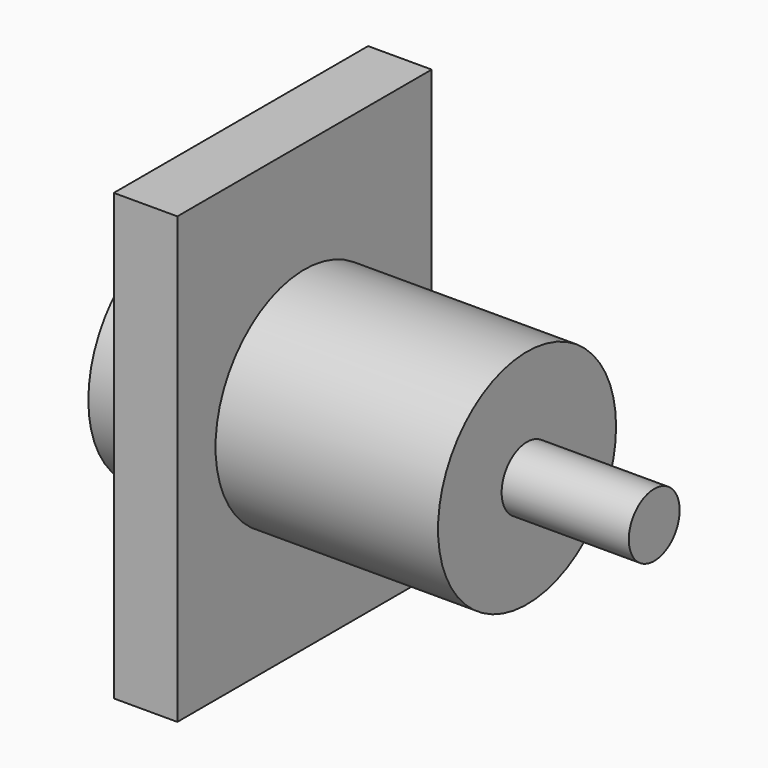
from build123d import *

# Parameters (mm, degrees)
F0_R     = 35
F1_DEPTH = 70
F2_R     = 10
F3_DEPTH = 40
F4_W     = 100
F4_H     = 140
F4_R     = 35
F5_DEPTH = 20
F6_R     = 35
F7_DEPTH = 20


with BuildPart() as f1:
    # F0 (on Right) → F1 (new body)
    with BuildSketch(Plane.YZ):
        Circle(F0_R)
    extrude(amount=F1_DEPTH)

    # F2 (on face) → F3 (join)
    with BuildSketch(Plane.YZ.offset(70)):
        Circle(F2_R)
    extrude(amount=F3_DEPTH)

    # F4 (on face) → F5 (join)
    with BuildSketch(Plane(origin=(0, 0, 0), x_dir=(0, -1, 0), z_dir=(-1, 0, 0))):
        Rectangle(F4_W, F4_H)
        Circle(F4_R, mode=Mode.SUBTRACT)
        Circle(F4_R)
    extrude(amount=F5_DEPTH)

    # F6 (on face) → F7 (join)
    with BuildSketch(Plane(origin=(-20, 0, 0), x_dir=(0, -1, 0), z_dir=(-1, 0, 0))):
        Circle(F6_R)
    extrude(amount=F7_DEPTH)


solid = f1.part
